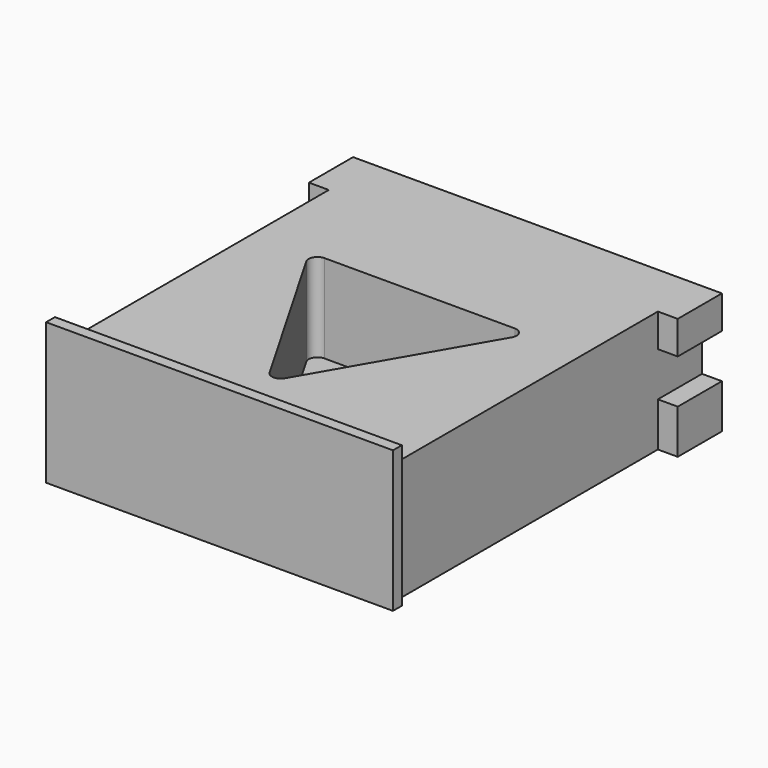
from build123d import *

# Parameters (mm, degrees)
F0_W     = 18.923
F0_H     = 6.985
F1_DEPTH = 22.86
F3_DEPTH = 0.635
F5_DEPTH = 5.08
F4_W     = 1.143
F4_H     = 3.175
F6_DEPTH = 6.985
F7_W     = 1.143
F7_H     = 2.54
F8_DEPTH = 12.7


# Not quite as in the source:
# - a feature names something its author has since deleted; it is built from what else it names


with BuildPart() as f1:
    # F0 (on Front) → F1 (new body)
    with BuildSketch(Plane.XZ):
        with Locations((0, -0.3175)):
            Rectangle(F0_W, F0_H)
    extrude(amount=F1_DEPTH)

    # F2 (on face) → F3 (join)
    with BuildSketch(Plane.XZ.offset(22.86)):
        Polygon((9.9764279214, 4.318), (-9.9695, 4.318), (-9.9695, -3.81), (-9.4615, -3.81), (-9.4615, 3.175), (9.4615, 3.175), (9.4615, -3.81), (9.9764279214, -3.81), align=None)
    extrude(amount=-F3_DEPTH)

    # F4 (on face) → F5 (cut)
    with BuildSketch(Plane.XY.offset(3.175)):
        with BuildLine():
            ThreePointArc((5.9100590949, -9.232738686), (5.9100590949, -8.724738686), (5.4701181898, -8.470738686))
            Line((5.4701181898, -8.470738686), (-5.4701181898, -8.470738686))
            ThreePointArc((-5.4701181898, -8.470738686), (-5.9100590949, -8.724738686), (-5.9100590949, -9.232738686))
            Line((-5.9100590949, -9.232738686), (-0.4399409051, -18.707261314))
            ThreePointArc((-0.4399409051, -18.707261314), (0, -18.961261314), (0.4399409051, -18.707261314))
            Line((0.4399409051, -18.707261314), (5.9100590949, -9.232738686))
        make_face()
    extrude(amount=-F5_DEPTH, mode=Mode.SUBTRACT)

    # F4 (on face) → F6 (join, through all)
    with BuildSketch(Plane.XY.offset(3.175)):
        with Locations((-10.033, -1.5875)):
            Rectangle(F4_W, F4_H)
        with Locations((10.033, -1.5875)):
            Rectangle(F4_W, F4_H)
    extrude(amount=-F6_DEPTH)

    # F7 (on face) → F8 (cut)
    with BuildSketch(Plane.XZ):
        with Locations((10.033, 0)):
            Rectangle(F7_W, F7_H)
        with Locations((-10.033, 0)):
            Rectangle(F7_W, F7_H)
    extrude(amount=F8_DEPTH, mode=Mode.SUBTRACT)


solid = f1.part
